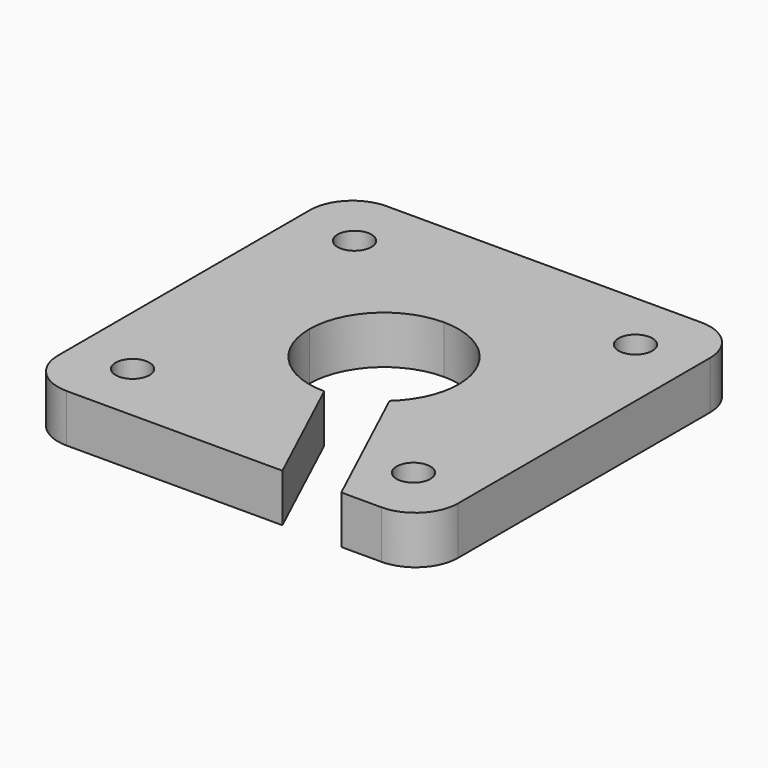
from build123d import *

# Parameters (mm, degrees)
F0_R     = 3.175
F1_DEPTH = 9


# Not quite as in the source:
# - ends of sketch curves that miss each other by under 0.0002 mm in the source are joined


with BuildPart() as f1:
    # F0 (on Top) → F1 (new body)
    with BuildSketch(Plane.XY):
        Polygon((10.95823, -37.5), (0, -14), (0, -37.5), align=None)
        with BuildLine():
            ThreePointArc((0, -14), (-9.8994949366, -9.8994949366), (-14, 0))
            Line((-14, 0), (-37.5, 0))
            Line((-37.5, 0), (-37.5, -29.5))
            ThreePointArc((-37.5, -29.5), (-35.1568542495, -35.1568542495), (-29.5, -37.5))
            Line((-29.5, -37.5), (0, -37.5))
            Line((0, -37.5), (0, -14))
        make_face()
        with Locations((-26.324893, -26)):
            Circle(F0_R, mode=Mode.SUBTRACT)
        with BuildLine():
            Line((37.5, 0), (14, 0))
            ThreePointArc((14, 0), (12.787539009, -5.6990215031), (9.3601648439, -10.4109228263))
            Line((9.3601648439, -10.4109228263), (21.992009, -37.5))
            Line((21.992009, -37.5), (29.5, -37.5))
            ThreePointArc((29.5, -37.5), (35.1568542495, -35.1568542495), (37.5, -29.5))
            Line((37.5, -29.5), (37.5, 0))
        make_face()
        with Locations((26.324893, -26)):
            Circle(F0_R, mode=Mode.SUBTRACT)
        with BuildLine():
            Line((29.5, 37.5), (0, 37.5))
            Line((0, 37.5), (0, 14))
            ThreePointArc((0, 14), (9.8994949366, 9.8994949366), (14, 0))
            Line((14, 0), (37.5, 0))
            Line((37.5, 0), (37.5, 29.5))
            ThreePointArc((37.5, 29.5), (35.1568542495, 35.1568542495), (29.5, 37.5))
        make_face()
        with Locations((26.324893, 26)):
            Circle(F0_R, mode=Mode.SUBTRACT)
        with BuildLine():
            Line((0, 14), (0, 37.5))
            Line((0, 37.5), (-29.5, 37.5))
            ThreePointArc((-29.5, 37.5), (-35.1568542495, 35.1568542495), (-37.5, 29.5))
            Line((-37.5, 29.5), (-37.5, 0))
            Line((-37.5, 0), (-14, 0))
            ThreePointArc((-14, 0), (-9.8994949366, 9.8994949366), (0, 14))
        make_face()
        with Locations((-26.324893, 26)):
            Circle(F0_R, mode=Mode.SUBTRACT)
    extrude(amount=F1_DEPTH)


solid = f1.part
